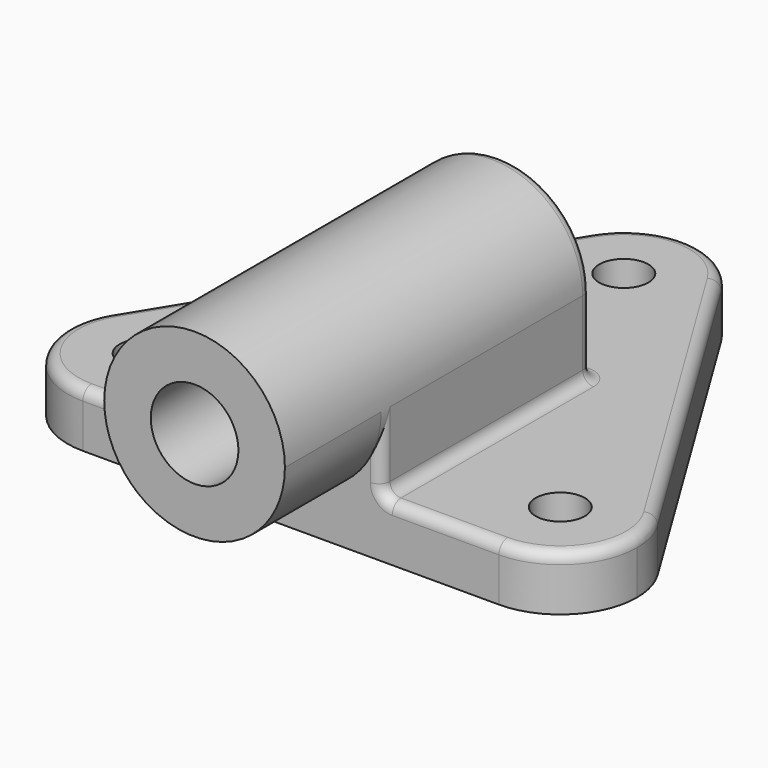
from build123d import *

# Parameters (mm, degrees)
F1_DEPTH     = 10
F3_DEPTH     = 22
F4_DEPTH     = 48
F6_D         = 16
F6_DEPTH     = 54
F6_TIP       = 4.8068849522
F7_T1_DEPTH  = 14
F7_T4_ANGLE  = 180
F7_T5_DEPTH  = 46
F7_T7_DEPTH  = 29
F7_T10_ANGLE = 90
F7_T12_ANGLE = 90
F7_T13_DEPTH = 19.5
F7_T15_DEPTH = 19.5
F7_T17_DEPTH = 72.7186358508
F7_T19_DEPTH = 72.7186358508
F7_T22_ANGLE = 121.5042667192
F7_T26_DEPTH = 20.5
F7_S27_R     = 16.5
F7_T28_DEPTH = 12
F7_T32_DEPTH = 20.5
F7_S33_R     = 16.5
F7_T34_DEPTH = 12
F7_T36_ANGLE = 121.5042667192
F7_T38_ANGLE = 116.9914665616
F7_T40_ANGLE = 90
F7_T42_ANGLE = 90
F9_D         = 9


# Not quite as in the source:
# - a fillet or chamfer that OpenCascade refuses, or shapes differently, is made with other operations: its cross-section is extruded or revolved along the edge and cut away or added


with BuildPart() as f1:
    # F0 (on Top) → F1 (new body)
    with BuildSketch(Plane.XY):
        with BuildLine():
            ThreePointArc((11.9364175338, 7.315868811), (13.4742318051, 3.8006680023), (14, 0))
            ThreePointArc((14, 0), (-3.8006680023, -13.4742318051), (-11.9364175338, 7.315868811))
            Line((-11.9364175338, 7.315868811), (-49.9364175338, -54.684131189))
            ThreePointArc((-49.9364175338, -54.684131189), (-34.1993319977, -48.5257681949), (-24, -62))
            ThreePointArc((-24, -62), (-28.1005050634, -71.8994949366), (-38, -76))
            Line((-38, -76), (38, -76))
            ThreePointArc((38, -76), (25.7848012019, -55.1597574368), (49.9364175338, -54.684131189))
            Line((49.9364175338, -54.684131189), (11.9364175338, 7.315868811))
        make_face()
        with BuildLine():
            ThreePointArc((-24, -62), (-34.1993319977, -48.5257681949), (-49.9364175338, -54.684131189))
            ThreePointArc((-49.9364175338, -54.684131189), (-50.2151987981, -68.8402425632), (-38, -76))
            ThreePointArc((-38, -76), (-28.1005050634, -71.8994949366), (-24, -62))
        make_face()
        with BuildLine():
            ThreePointArc((-11.9364175338, 7.315868811), (-3.8006680023, -13.4742318051), (14, 0))
            ThreePointArc((14, 0), (13.4742318051, 3.8006680023), (11.9364175338, 7.315868811))
            ThreePointArc((11.9364175338, 7.315868811), (0, 14), (-11.9364175338, 7.315868811))
        make_face()
        with BuildLine():
            ThreePointArc((52, -62), (51.4742318051, -58.1993319977), (49.9364175338, -54.684131189))
            ThreePointArc((49.9364175338, -54.684131189), (25.7848012019, -55.1597574368), (38, -76))
            ThreePointArc((38, -76), (47.8994949366, -71.8994949366), (52, -62))
        make_face()
    extrude(amount=F1_DEPTH)

    # F2 (on face) → F3 (join)
    with BuildSketch(Plane.XZ.offset(76)):
        with BuildLine():
            ThreePointArc((8.7321245983, 10), (14.4279252818, 15.9946910076), (16.5, 24))
            ThreePointArc((16.5, 24), (0, 40.5), (-16.5, 24))
            ThreePointArc((-16.5, 24), (-14.4279252818, 15.9946910076), (-8.7321245983, 10))
            Line((-8.7321245983, 10), (8.7321245983, 10))
        make_face()
        with BuildLine():
            ThreePointArc((-8.7321245983, 10), (0, 7.5), (8.7321245983, 10))
            Line((8.7321245983, 10), (-8.7321245983, 10))
        make_face()
    extrude(amount=F3_DEPTH)

    # F2 (on face) → F4 (join)
    with BuildSketch(Plane.XZ.offset(76)):
        with BuildLine():
            Line((16.5, 10), (16.5, 24))
            ThreePointArc((16.5, 24), (14.4279252818, 15.9946910076), (8.7321245983, 10))
            Line((8.7321245983, 10), (16.5, 10))
        make_face()
        with BuildLine():
            ThreePointArc((8.7321245983, 10), (14.4279252818, 15.9946910076), (16.5, 24))
            ThreePointArc((16.5, 24), (0, 40.5), (-16.5, 24))
            ThreePointArc((-16.5, 24), (-14.4279252818, 15.9946910076), (-8.7321245983, 10))
            Line((-8.7321245983, 10), (8.7321245983, 10))
        make_face()
        with BuildLine():
            ThreePointArc((-8.7321245983, 10), (-14.4279252818, 15.9946910076), (-16.5, 24))
            Line((-16.5, 24), (-16.5, 10))
            Line((-16.5, 10), (-8.7321245983, 10))
        make_face()
    extrude(amount=-F4_DEPTH)

    # F6
    with Locations(Plane.XZ.offset(98)):
        with Locations((0, 24)):
            Hole(F6_D / 2, depth=F6_DEPTH)
            with Locations((0, 0, -(F6_DEPTH + F6_TIP / 2))):  # 118° drill point
                Cone(0, F6_D / 2, F6_TIP, mode=Mode.SUBTRACT)

    # F7: fillet of radius 2 on 15 edges, made by hand

    # F7_s2 → F7_t1 (cut)
    with BuildSketch(Plane.XY.offset(10)):
        with BuildLine():
            ThreePointArc((-16.5, -30), (-15.9142135624, -28.5857864376), (-14.5, -28))
            Line((-14.5, -28), (-16.5, -28))
            Line((-16.5, -28), (-16.5, -30))
        make_face()
        with BuildLine():
            ThreePointArc((16.5, -30), (15.9142135624, -28.5857864376), (14.5, -28))
            Line((14.5, -28), (16.5, -28))
            Line((16.5, -28), (16.5, -30))
        make_face()
    extrude(amount=F7_T1_DEPTH, mode=Mode.SUBTRACT)

    # F7_s3 → F7_t4 (revolve, cut)
    with BuildSketch(Plane.XY.offset(24)):
        with BuildLine():
            ThreePointArc((16.5, -30), (15.9142135624, -28.5857864376), (14.5, -28))
            Line((14.5, -28), (16.5, -28))
            Line((16.5, -28), (16.5, -30))
        make_face()
    revolve(axis=Axis((0, -28, 24), (0, -1, 0)), revolution_arc=F7_T4_ANGLE, mode=Mode.SUBTRACT)

    # F7_s6 → F7_t5 (join)
    with BuildSketch(Plane.XZ.offset(30)):
        with BuildLine():
            ThreePointArc((18.5, 10), (17.0857864376, 10.5857864376), (16.5, 12))
            Line((16.5, 12), (16.5, 10))
            Line((16.5, 10), (18.5, 10))
        make_face()
        with BuildLine():
            ThreePointArc((-18.5, 10), (-17.0857864376, 10.5857864376), (-16.5, 12))
            Line((-16.5, 12), (-16.5, 10))
            Line((-16.5, 10), (-18.5, 10))
        make_face()
    extrude(amount=F7_T5_DEPTH)

    # F7_s8 → F7_t7 (join)
    with BuildSketch(Plane.YZ.offset(-14.5)):
        with BuildLine():
            ThreePointArc((-26, 10), (-27.4142135624, 10.5857864376), (-28, 12))
            Line((-28, 12), (-28, 10))
            Line((-28, 10), (-26, 10))
        make_face()
    extrude(amount=F7_T7_DEPTH)

    # F7_s9 → F7_t10 (revolve)
    with BuildSketch(Plane.XZ.offset(30)):
        with BuildLine():
            ThreePointArc((-18.5, 10), (-17.0857864376, 10.5857864376), (-16.5, 12))
            Line((-16.5, 12), (-16.5, 10))
            Line((-16.5, 10), (-18.5, 10))
        make_face()
    revolve(axis=Axis((-14.5, -30, 10), (0, 0, -1)), revolution_arc=F7_T10_ANGLE)

    # F7_s11 → F7_t12 (revolve)
    with BuildSketch(Plane.XZ.offset(30)):
        with BuildLine():
            ThreePointArc((18.5, 10), (17.0857864376, 10.5857864376), (16.5, 12))
            Line((16.5, 12), (16.5, 10))
            Line((16.5, 10), (18.5, 10))
        make_face()
    revolve(axis=Axis((14.5, -30, 10), (0, 0, 1)), revolution_arc=F7_T12_ANGLE)

    # F7_s14 → F7_t13 (cut)
    with BuildSketch(Plane.YZ.offset(-38)):
        with BuildLine():
            ThreePointArc((-76, 8), (-75.4142135624, 9.4142135624), (-74, 10))
            Line((-74, 10), (-76, 10))
            Line((-76, 10), (-76, 8))
        make_face()
    extrude(amount=F7_T13_DEPTH, mode=Mode.SUBTRACT)

    # F7_s16 → F7_t15 (cut)
    with BuildSketch(Plane.YZ.offset(18.5)):
        with BuildLine():
            ThreePointArc((-76, 8), (-75.4142135624, 9.4142135624), (-74, 10))
            Line((-74, 10), (-76, 10))
            Line((-76, 10), (-76, 8))
        make_face()
    extrude(amount=F7_T15_DEPTH, mode=Mode.SUBTRACT)

    # F7_s18 → F7_t17 (cut)
    with BuildSketch(Plane(origin=(0, 0, 0), x_dir=(0, 0, 1), z_dir=(-0.5225620579, -0.8526012524, 0))):
        with BuildLine():
            ThreePointArc((10, 12), (9.4142135624, 13.4142135624), (8, 14))
            Line((8, 14), (10, 14))
            Line((10, 14), (10, 12))
        make_face()
    extrude(amount=F7_T17_DEPTH, mode=Mode.SUBTRACT)

    # F7_s20 → F7_t19 (cut)
    with BuildSketch(Plane(origin=(38, -62, 0), x_dir=(0, 0, 1), z_dir=(-0.5225620579, 0.8526012524, 0))):
        with BuildLine():
            ThreePointArc((10, 12), (9.4142135624, 13.4142135624), (8, 14))
            Line((8, 14), (10, 14))
            Line((10, 14), (10, 12))
        make_face()
    extrude(amount=F7_T19_DEPTH, mode=Mode.SUBTRACT)

    # F7_s21 → F7_t22 (revolve, cut)
    with BuildSketch(Plane.YZ.offset(38)):
        with BuildLine():
            ThreePointArc((-74, 10), (-75.4142135624, 9.4142135624), (-76, 8))
            Line((-76, 8), (-76, 10))
            Line((-76, 10), (-74, 10))
        make_face()
    revolve(axis=Axis((38, -62, 10), (0, 0, 1)), revolution_arc=F7_T22_ANGLE, mode=Mode.SUBTRACT)


with BuildPart() as f7_tool24:
    # F7_s25 → F7_t26 (new body)
    with BuildSketch(Plane.XY.offset(12)):
        with BuildLine():
            ThreePointArc((14.5, -76), (15.9142135624, -75.4142135624), (16.5, -74))
            Line((16.5, -74), (16.5, -76))
            Line((16.5, -76), (14.5, -76))
        make_face()
    extrude(amount=F7_T26_DEPTH)

    # F7_s27 → F7_t28 (cut, symmetric)
    with BuildSketch(Plane.XZ.offset(75)):
        with Locations((0, 24)):
            Circle(F7_S27_R)
    extrude(amount=F7_T28_DEPTH, both=True, mode=Mode.SUBTRACT)


with BuildPart() as f1_1:
    add(f1.part)

    # F7_t23: cut F7_tool24
    add(f7_tool24.part, mode=Mode.SUBTRACT)


with BuildPart() as f7_tool30:
    # F7_s31 → F7_t32 (new body)
    with BuildSketch(Plane.XY.offset(32.5)):
        with BuildLine():
            ThreePointArc((-14.5, -76), (-15.9142135624, -75.4142135624), (-16.5, -74))
            Line((-16.5, -74), (-16.5, -76))
            Line((-16.5, -76), (-14.5, -76))
        make_face()
    extrude(amount=-F7_T32_DEPTH)

    # F7_s33 → F7_t34 (cut, symmetric)
    with BuildSketch(Plane.XZ.offset(75)):
        with Locations((0, 24)):
            Circle(F7_S33_R)
    extrude(amount=F7_T34_DEPTH, both=True, mode=Mode.SUBTRACT)


with BuildPart() as f1_2:
    add(f1_1.part)

    # F7_t29: cut F7_tool30
    add(f7_tool30.part, mode=Mode.SUBTRACT)

    # F7_s35 → F7_t36 (revolve, cut)
    with BuildSketch(Plane(origin=(-38, -62, 0), x_dir=(0, 0, 1), z_dir=(0.5225620579, 0.8526012524, 0))):
        with BuildLine():
            ThreePointArc((8, -14), (9.4142135624, -13.4142135624), (10, -12))
            Line((10, -12), (10, -14))
            Line((10, -14), (8, -14))
        make_face()
    revolve(axis=Axis((-38, -62, 10), (0, 0, 1)), revolution_arc=F7_T36_ANGLE, mode=Mode.SUBTRACT)

    # F7_s37 → F7_t38 (revolve, cut)
    with BuildSketch(Plane(origin=(0, 0, 0), x_dir=(0, 0, 1), z_dir=(0.5225620579, -0.8526012524, 0))):
        with BuildLine():
            ThreePointArc((10, -12), (9.4142135624, -13.4142135624), (8, -14))
            Line((8, -14), (10, -14))
            Line((10, -14), (10, -12))
        make_face()
    revolve(axis=Axis((0, 0, 10), (0, 0, 1)), revolution_arc=F7_T38_ANGLE, mode=Mode.SUBTRACT)

    # F7_s39 → F7_t40 (revolve, cut)
    with BuildSketch(Plane.YZ.offset(18.5)):
        with BuildLine():
            ThreePointArc((-76, 8), (-75.4142135624, 9.4142135624), (-74, 10))
            Line((-74, 10), (-76, 10))
            Line((-76, 10), (-76, 8))
        make_face()
    revolve(axis=Axis((18.5, -76, 12), (0, 1, 0)), revolution_arc=F7_T40_ANGLE, mode=Mode.SUBTRACT)

    # F7_s41 → F7_t42 (revolve, cut)
    with BuildSketch(Plane.YZ.offset(-18.5)):
        with BuildLine():
            ThreePointArc((-76, 8), (-75.4142135624, 9.4142135624), (-74, 10))
            Line((-74, 10), (-76, 10))
            Line((-76, 10), (-76, 8))
        make_face()
    revolve(axis=Axis((-18.5, -76, 12), (0, -1, 0)), revolution_arc=F7_T42_ANGLE, mode=Mode.SUBTRACT)

    # F9 (through all)
    with Locations(Plane.XY.offset(10)):
        with Locations((38, -62), (0, 0), (-38, -62)):
            Hole(F9_D / 2)


solid = f1_2.part
